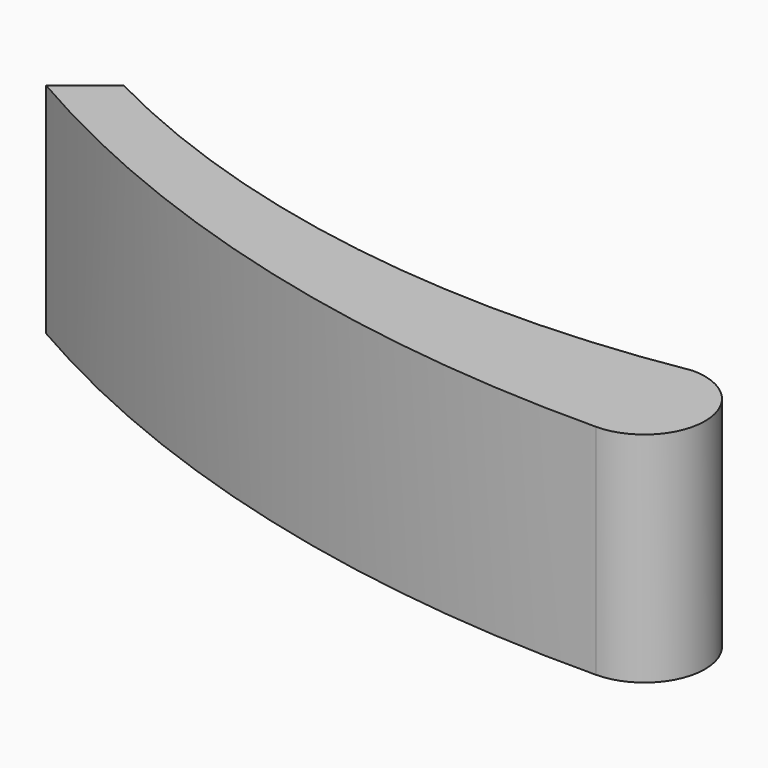
from build123d import *

# Parameters (mm, degrees)
F1_DEPTH = 45.72


# Not quite as in the source:
# - a feature of the source that left no trace in its solid (it failed there, or was rolled back) is left out


with BuildPart() as f1:
    # F0 (on Top) → F1 (new body)
    with BuildSketch(Plane.XY):
        with BuildLine():
            ThreePointArc((-145.6707853291, 26.9605556957), (-75.3977689013, -1.915708772), (0, -11.2597941826))
            ThreePointArc((0, -11.2597941826), (12.7, 1.4402058174), (0, 14.1402058174))
            ThreePointArc((0, 14.1402058174), (-69.5452300972, 13.4738928601), (-135.7246581581, 34.8576788616))
            Line((-135.7246581581, 34.8576788616), (-145.6707853291, 26.9605556957))
        make_face()
    extrude(amount=F1_DEPTH)


solid = f1.part
